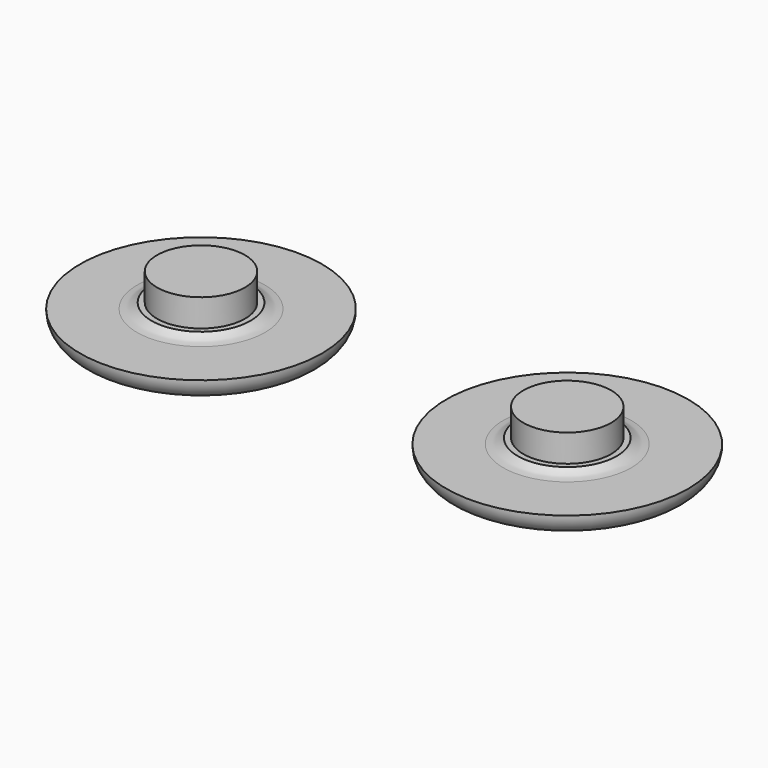
from build123d import *

# Parameters (mm, degrees)
F0_R         = 11
F1_DEPTH     = 2
F2_R         = 4.5
F3_DEPTH     = 0.5
F4_R         = 3.995
F5_DEPTH     = 2.5
F7_TEXT_SIZE = 6.9444444444
F10_DEPTH    = 1
F9_TEXT_SIZE = 3.75
F11_DEPTH    = 1


# Not quite as in the source:
# - a fillet or chamfer that OpenCascade refuses, or shapes differently, is made with other operations: its cross-section is extruded or revolved along the edge and cut away or added
# - Text() gives the source's letters only with a copy of the font that has no kerning and outlines rounded to 1/6400 em; it was checked with that copy


with BuildPart() as f1:
    # F0 (on Top) → F1 (new body)
    with BuildSketch(Plane.XY):
        with Locations((-124.7583553195, 13.61318212)):
            Circle(F0_R)
    extrude(amount=F1_DEPTH)

    # F2 (on face) → F3 (join)
    with BuildSketch(Plane.XY.offset(2)):
        with Locations((-124.7583553195, 13.61318212)):
            Circle(F2_R)
    extrude(amount=F3_DEPTH)

    # F4 (on face) → F5 (join)
    with BuildSketch(Plane.XY.offset(2.5)):
        with Locations((-124.7583553195, 13.61318212)):
            Circle(F4_R)
    extrude(amount=F5_DEPTH)

    # F6: fillet of radius 2 on 2 edges, made by hand

    # F6_s1 → F6_t2 (revolve)
    with BuildSketch(Plane.XZ.offset(-13.61318212)):
        with BuildLine():
            ThreePointArc((-118.935479664, 2), (-119.6425864452, 2.1291713066), (-120.2583553195, 2.5))
            Line((-120.2583553195, 2.5), (-120.2583553195, 2))
            Line((-120.2583553195, 2), (-118.935479664, 2))
        make_face()
    revolve(axis=Axis((-124.7583553195, 13.61318212, 2), (0, 0, 1)))

    # F6_s3 → F6_t4 (revolve, cut)
    with BuildSketch(Plane.XZ.offset(-13.61318212)):
        with BuildLine():
            ThreePointArc((-113.7583553195, 2), (-114.3441417571, 0.5857864376), (-115.7583553195, 0))
            Line((-115.7583553195, 0), (-113.7583553195, 0))
            Line((-113.7583553195, 0), (-113.7583553195, 2))
        make_face()
    revolve(axis=Axis((-124.7583553195, 13.61318212, 0), (0, 0, 1)), mode=Mode.SUBTRACT)


with BuildPart() as f8_1:
    # F8: copy of F1
    add(f1.part.moved(Location((33.3, 0, 0))))

    # F9 (on face) → F11 (cut)
    with BuildSketch(Plane(origin=(0, 0, 0), x_dir=(1, 0, 0), z_dir=(0, 0, -1))):
        with Locations((-98.0938435316, -11.6118247434)):
            Text('sawyer', F9_TEXT_SIZE, font='Open Sans', font_style=FontStyle.BOLD, text_align=(TextAlign.LEFT, TextAlign.BOTTOM))
        with Locations((-99.0682575941, -16.7118247434)):
            Text('spinners', F9_TEXT_SIZE, font='Open Sans', font_style=FontStyle.BOLD, text_align=(TextAlign.LEFT, TextAlign.BOTTOM))
    extrude(amount=-F11_DEPTH, mode=Mode.SUBTRACT)


with BuildPart() as f1_1:
    add(f1.part)

    # F7 (on face) → F10 (cut)
    with BuildSketch(Plane(origin=(0, 0, 0), x_dir=(1, 0, 0), z_dir=(0, 0, -1))):
        with Locations((-131.5992479987, -15.816334672)):
            Text('c8/9', F7_TEXT_SIZE, font='Open Sans', text_align=(TextAlign.LEFT, TextAlign.BOTTOM))
    extrude(amount=-F10_DEPTH, mode=Mode.SUBTRACT)


solid = Compound([f8_1.part, f1_1.part])
